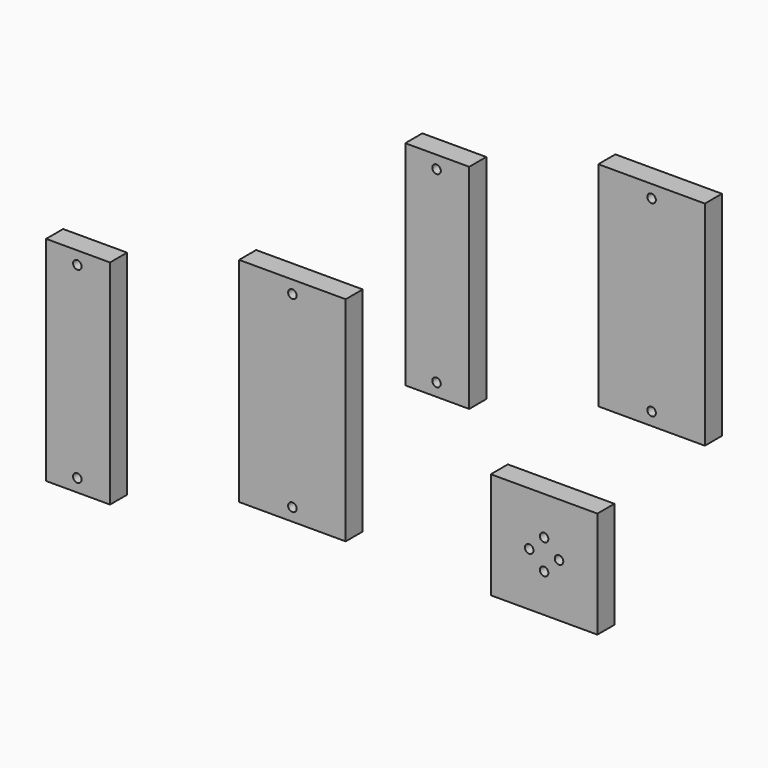
from build123d import *

# Parameters (mm, degrees)
F0_W     = 15
F0_H     = 50
F0_R     = 1
F1_DEPTH = 5
F2_DEPTH = 5
F0_W_2   = 25
F0_H_2   = 25


# Not quite as in the source:
# - a feature names something its author has since deleted; it is built from what else it names


with BuildPart() as f1:
    # F0 (on Front) → F1 (new body)
    with BuildSketch(Plane.XZ):
        with Locations((0.1666661408, 25)):
            Rectangle(F0_W, F0_H)
        with Locations((0, 3)):
            Circle(F0_R, mode=Mode.SUBTRACT)
        with Locations((0, 47)):
            Circle(F0_R, mode=Mode.SUBTRACT)
    extrude(amount=F1_DEPTH)

    # F0 (on Front) → F2 (join)
    with BuildSketch(Plane.XZ):
        with Locations((0.1666661408, 25)):
            Rectangle(F0_W, F0_H)
        with Locations((0, 3)):
            Circle(F0_R, mode=Mode.SUBTRACT)
        with Locations((0, 47)):
            Circle(F0_R, mode=Mode.SUBTRACT)
    extrude(amount=F2_DEPTH)


with BuildPart() as f2:
    # F0 (on Front) → F2, piece 2 (new body)
    with BuildSketch(Plane.XZ):
        with Locations((50.4353579649, 35.3805905879)):
            Rectangle(F0_W_2, F0_H)
        with Locations((50.4353579649, 13.3805905879)):
            Circle(F0_R, mode=Mode.SUBTRACT)
        with Locations((50.4353579649, 57.3805905879)):
            Circle(F0_R, mode=Mode.SUBTRACT)
    extrude(amount=F2_DEPTH)


with BuildPart() as f2b:
    # F0 (on Front) → F2, piece 3 (new body)
    with BuildSketch(Plane.XZ):
        with Locations((-84.0754437791, -22.1488411874)):
            Rectangle(F0_W, F0_H)
        with Locations((-84.2421099199, -44.1488411874)):
            Circle(F0_R, mode=Mode.SUBTRACT)
        with Locations((-84.2421099199, -0.1488411874)):
            Circle(F0_R, mode=Mode.SUBTRACT)
    extrude(amount=F2_DEPTH)


with BuildPart() as f2c:
    # F0 (on Front) → F2, piece 4 (new body)
    with BuildSketch(Plane.XZ):
        with Locations((-33.806751955, -11.7682505995)):
            Rectangle(F0_W_2, F0_H)
        with Locations((-33.806751955, -33.7682505995)):
            Circle(F0_R, mode=Mode.SUBTRACT)
        with Locations((-33.806751955, 10.2317494005)):
            Circle(F0_R, mode=Mode.SUBTRACT)
    extrude(amount=F2_DEPTH)


with BuildPart() as f2d:
    # F0 (on Front) → F2, piece 5 (new body)
    with BuildSketch(Plane.XZ):
        with Locations((25.2282431349, -24.3284247816)):
            Rectangle(F0_W_2, F0_H_2)
        with Locations((21.7282431349, -24.3284247816)):
            Circle(F0_R, mode=Mode.SUBTRACT)
        with Locations((25.2282431349, -27.8284247816)):
            Circle(F0_R, mode=Mode.SUBTRACT)
        with Locations((28.7282431349, -24.3284247816)):
            Circle(F0_R, mode=Mode.SUBTRACT)
        with Locations((25.2282431349, -20.8284247816)):
            Circle(F0_R, mode=Mode.SUBTRACT)
    extrude(amount=F2_DEPTH)


solid = Compound([f1.part, f2.part, f2b.part, f2c.part, f2d.part])
